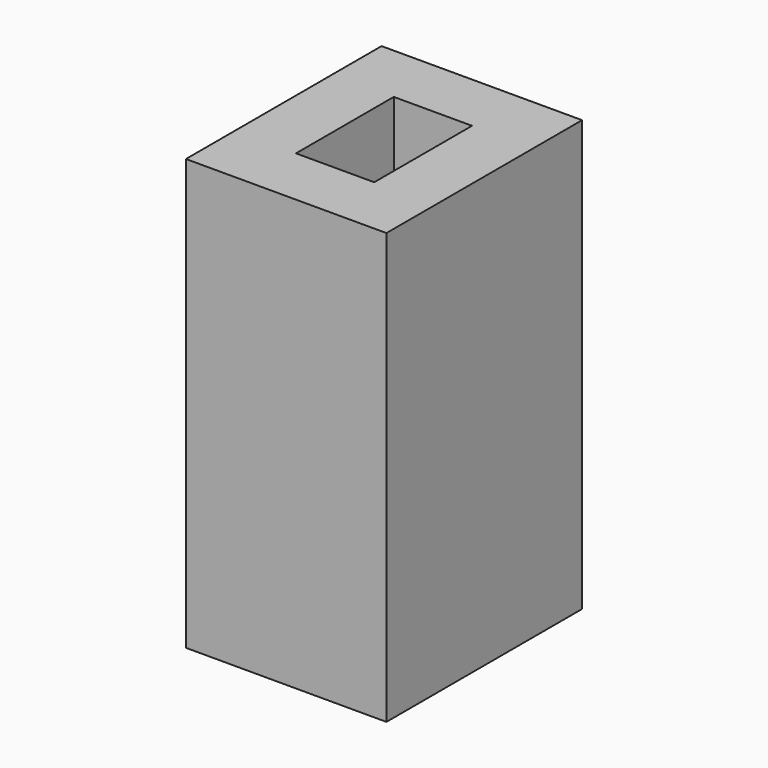
from build123d import *

# Parameters (mm, degrees)
F0_W     = 8.2
F0_H     = 10
F0_W_2   = 3.2
F0_H_2   = 5
F1_DEPTH = 17.6


# Not quite as in the source:
# - a feature names something its author has since deleted; it is built from what else it names


with BuildPart() as f1:
    # F0 (on Top) → F1 (new body)
    with BuildSketch(Plane.XY):
        with Locations((-15.9300868601, 0.8088900894)):
            Rectangle(F0_W, F0_H)
        with Locations((-15.9300868601, 0.8088900894)):
            Rectangle(F0_W_2, F0_H_2, mode=Mode.SUBTRACT)
    extrude(amount=F1_DEPTH)


solid = f1.part
